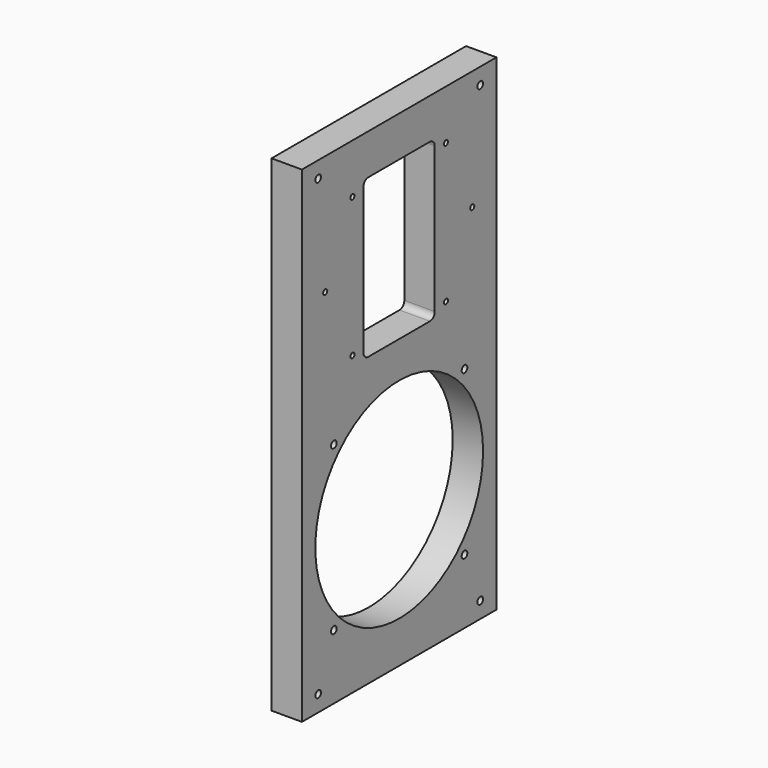
from build123d import *

# Parameters (mm, degrees)
F0_W     = 120
F0_H     = 240
F0_R     = 1.75
F0_R_2   = 51.75
F0_R_3   = 1.25
F1_DEPTH = 15


# Not quite as in the source:
# - a feature names something its author has since deleted; it is built from what else it names


with BuildPart() as f1:
    # F0 (on Right) → F1 (new body)
    with BuildSketch(Plane.YZ):
        with Locations((0, 4.9354011911)):
            Rectangle(F0_W, F0_H)
        with Locations((-49.9999973178, -107.0645988089)):
            Circle(F0_R, mode=Mode.SUBTRACT)
        with Locations((-40.3050865276, -83.1196853366)):
            Circle(F0_R, mode=Mode.SUBTRACT)
        with Locations((-40.3050865276, -2.5095122813)):
            Circle(F0_R, mode=Mode.SUBTRACT)
        with Locations((50.0000026822, -107.0645988089)):
            Circle(F0_R, mode=Mode.SUBTRACT)
        with Locations((40.3050865276, -83.1196853366)):
            Circle(F0_R, mode=Mode.SUBTRACT)
        with Locations((0, -42.8145988089)):
            Circle(F0_R_2, mode=Mode.SUBTRACT)
        with Locations((40.3050865276, -2.5095122813)):
            Circle(F0_R, mode=Mode.SUBTRACT)
        with Locations((-28.8463527312, 31.4634012507)):
            Circle(F0_R_3, mode=Mode.SUBTRACT)
        with Locations((-45.6305965781, 65.8711940348)):
            Circle(F0_R_3, mode=Mode.SUBTRACT)
        with Locations((-49.9999973178, 116.9354011911)):
            Circle(F0_R, mode=Mode.SUBTRACT)
        with BuildLine():
            ThreePointArc((-22.0790897047, 101.9354011911), (-21.2004100483, 104.0567215346), (-19.0790897047, 104.9354011911))
            Line((-19.0790897047, 104.9354011911), (18.9209102953, 104.9354011911))
            ThreePointArc((18.9209102953, 104.9354011911), (21.0422306388, 104.0567215346), (21.9209102953, 101.9354011911))
            Line((21.9209102953, 101.9354011911), (21.9209102953, 29.9354011911))
            ThreePointArc((21.9209102953, 29.9354011911), (21.0422306388, 27.8140808475), (18.9209102953, 26.9354011911))
            Line((18.9209102953, 26.9354011911), (-19.0790897047, 26.9354011911))
            ThreePointArc((-19.0790897047, 26.9354011911), (-21.2004100483, 27.8140808475), (-22.0790897047, 29.9354011911))
            Line((-22.0790897047, 29.9354011911), (-22.0790897047, 101.9354011911))
        make_face(mode=Mode.SUBTRACT)
        with Locations((-28.8463527312, 100.4074011314)):
            Circle(F0_R_3, mode=Mode.SUBTRACT)
        with Locations((28.8463527312, 31.4634012507)):
            Circle(F0_R_3, mode=Mode.SUBTRACT)
        with Locations((28.8463527312, 100.4074011314)):
            Circle(F0_R_3, mode=Mode.SUBTRACT)
        with Locations((45.0773127377, 65.8711940348)):
            Circle(F0_R_3, mode=Mode.SUBTRACT)
        with Locations((50.0000026822, 116.9354046481)):
            Circle(F0_R, mode=Mode.SUBTRACT)
    extrude(amount=-F1_DEPTH)


solid = f1.part
